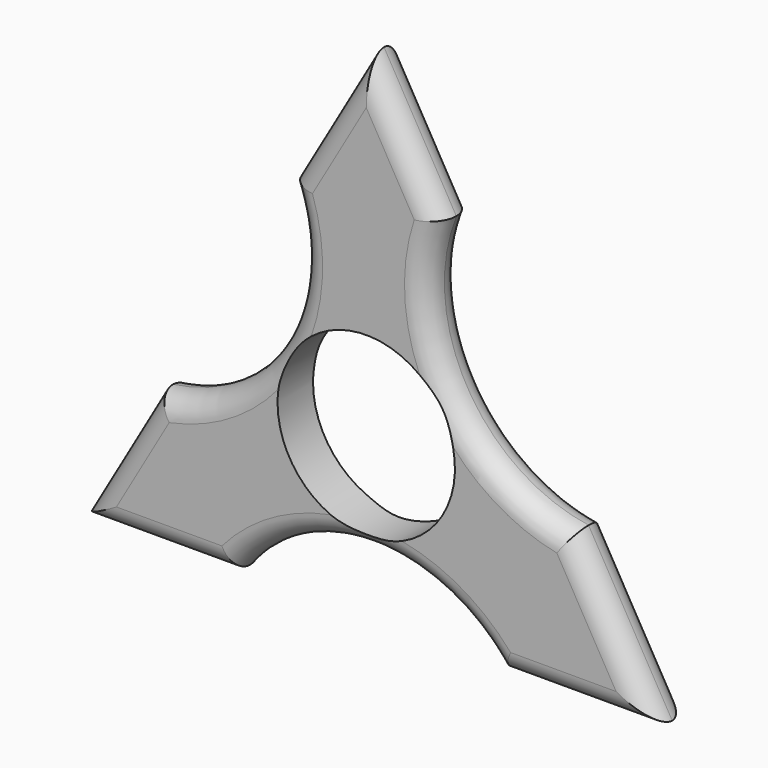
from build123d import *

# Parameters (mm, degrees)
F2_DEPTH     = 5
F3_D         = 20
F5_DEPTH     = 5
F7_T1_DEPTH  = 28.8144071543
F7_T3_DEPTH  = 30.1295341717
F7_T5_DEPTH  = 31.3559112982
F7_T7_DEPTH  = 29.9091460928
F7_T9_DEPTH  = 29.9091460928
F7_T11_DEPTH = 29.9018260823
F7_T14_ANGLE = 141.1544022781
F7_T16_ANGLE = 142.8852494642
F7_T18_ANGLE = 141.8336244917
F7_T20_ANGLE = 141.8336244917
F7_T22_ANGLE = 141.1544022781
F7_T24_ANGLE = 142.8852494642


# Not quite as in the source:
# - a fillet or chamfer that OpenCascade refuses, or shapes differently, is made with other operations: its cross-section is extruded or revolved along the edge and cut away or added
# - a feature of the source that left no trace in its solid (it failed there, or was rolled back) is left out


with BuildPart() as f2:
    # F0 (on Front) → F2 (new body)
    with BuildSketch(Plane.XZ):
        Polygon((0, 56.291651246), (-32.5, 0), (32.5, 0), align=None)
    extrude(amount=F2_DEPTH)

    # F3 (through all)
    with Locations(Plane(origin=(0, 0, 0), x_dir=(1, 0, 0), z_dir=(0, 1, 0))):
        with Locations((0, -18.7304634601)):
            Hole(F3_D / 2)

    # F4 (on face) → F5 (cut)
    with BuildSketch(Plane.XZ.offset(5)):
        with BuildLine():
            Line((-8.8147670858, 41.0240267964), (-23.7990869589, 15.0704234595))
            ThreePointArc((-23.7990869589, 15.0704234595), (-9.9693914422, 24.3882472548), (-8.8147670858, 41.0240267964))
        make_face()
        with BuildLine():
            Line((23.0720443509, 16.3296981957), (8.1572035772, 42.1629602027))
            ThreePointArc((8.1572035772, 42.1629602027), (9.353798316, 25.631639826), (23.0720443509, 16.3296981957))
        make_face()
        with BuildLine():
            ThreePointArc((15.0908539072, 0), (0, 7.455905044), (-15.0908539072, 0))
            Line((-15.0908539072, 0), (15.0908539072, 0))
        make_face()
    extrude(amount=-F5_DEPTH, mode=Mode.SUBTRACT)

    # F7: fillet of radius 2.5 on 18 edges, made by hand

    # F7_s2 → F7_t1 (cut)
    with BuildSketch(Plane(origin=(-13.0927964228, 0, 22.6773886175), x_dir=(0, 1, 0), z_dir=(-0.5, 0, 0.8660254038))):
        with BuildLine():
            ThreePointArc((0, -25.645825623), (-0.732233047, -27.413592576), (-2.5, -28.145825623))
            Line((-2.5, -28.145825623), (0, -28.145825623))
            Line((0, -28.145825623), (0, -25.645825623))
        make_face()
        with BuildLine():
            ThreePointArc((-5, -25.645825623), (-4.267766953, -27.413592576), (-2.5, -28.145825623))
            Line((-2.5, -28.145825623), (-5, -28.145825623))
            Line((-5, -28.145825623), (-5, -25.645825623))
        make_face()
    extrude(amount=F7_T1_DEPTH, mode=Mode.SUBTRACT)

    # F7_s4 → F7_t3 (cut)
    with BuildSketch(Plane(origin=(27.5, 0, 47.6313972081), x_dir=(0, 1, 0), z_dir=(-0.5, 0, -0.8660254038))):
        with BuildLine():
            ThreePointArc((-2.5, -28.145825623), (-0.732233047, -27.413592576), (0, -25.645825623))
            Line((0, -25.645825623), (0, -28.145825623))
            Line((0, -28.145825623), (-2.5, -28.145825623))
        make_face()
        with BuildLine():
            ThreePointArc((-2.5, -28.145825623), (-4.267766953, -27.413592576), (-5, -25.645825623))
            Line((-5, -25.645825623), (-5, -28.145825623))
            Line((-5, -28.145825623), (-2.5, -28.145825623))
        make_face()
    extrude(amount=F7_T3_DEPTH, mode=Mode.SUBTRACT)

    # F7_s6 → F7_t5 (cut)
    with BuildSketch(Plane(origin=(11.25, 0, -19.4855715851), x_dir=(0, 1, 0), z_dir=(-0.5, 0, 0.8660254038))):
        with BuildLine():
            ThreePointArc((0, -25.645825623), (-0.732233047, -27.413592576), (-2.5, -28.145825623))
            Line((-2.5, -28.145825623), (0, -28.145825623))
            Line((0, -28.145825623), (0, -25.645825623))
        make_face()
        with BuildLine():
            ThreePointArc((-5, -25.645825623), (-4.267766953, -27.413592576), (-2.5, -28.145825623))
            Line((-2.5, -28.145825623), (-5, -28.145825623))
            Line((-5, -28.145825623), (-5, -25.645825623))
        make_face()
    extrude(amount=F7_T5_DEPTH, mode=Mode.SUBTRACT)

    # F7_s8 → F7_t7 (cut)
    with BuildSketch(Plane.YZ.offset(8.8408539072)):
        with BuildLine():
            ThreePointArc((0, 2.5), (-0.732233047, 0.732233047), (-2.5, 0))
            Line((-2.5, 0), (0, 0))
            Line((0, 0), (0, 2.5))
        make_face()
        with BuildLine():
            ThreePointArc((-5, 2.5), (-4.267766953, 0.732233047), (-2.5, 0))
            Line((-2.5, 0), (-5, 0))
            Line((-5, 0), (-5, 2.5))
        make_face()
    extrude(amount=F7_T7_DEPTH, mode=Mode.SUBTRACT)

    # F7_s10 → F7_t9 (cut)
    with BuildSketch(Plane.YZ.offset(-38.75)):
        with BuildLine():
            ThreePointArc((0, 2.5), (-0.732233047, 0.732233047), (-2.5, 0))
            Line((-2.5, 0), (0, 0))
            Line((0, 0), (0, 2.5))
        make_face()
        with BuildLine():
            ThreePointArc((-5, 2.5), (-4.267766953, 0.732233047), (-2.5, 0))
            Line((-2.5, 0), (-5, 0))
            Line((-5, 0), (-5, 2.5))
        make_face()
    extrude(amount=F7_T9_DEPTH, mode=Mode.SUBTRACT)

    # F7_s12 → F7_t11 (cut)
    with BuildSketch(Plane(origin=(3.7009130411, 0, 6.4101694217), x_dir=(0, 1, 0), z_dir=(-0.5, 0, -0.8660254038))):
        with BuildLine():
            ThreePointArc((0, -25.645825623), (-0.732233047, -27.413592576), (-2.5, -28.145825623))
            Line((-2.5, -28.145825623), (0, -28.145825623))
            Line((0, -28.145825623), (0, -25.645825623))
        make_face()
        with BuildLine():
            ThreePointArc((-5, -25.645825623), (-4.267766953, -27.413592576), (-2.5, -28.145825623))
            Line((-2.5, -28.145825623), (-5, -28.145825623))
            Line((-5, -28.145825623), (-5, -25.645825623))
        make_face()
    extrude(amount=F7_T11_DEPTH, mode=Mode.SUBTRACT)

    # F7_s13 → F7_t14 (revolve, cut)
    with BuildSketch(Plane(origin=(28.2767394092, 0, 33.0176183098), x_dir=(0, 1, 0), z_dir=(0.6504720402, 0, 0.7595302002))):
        with BuildLine():
            ThreePointArc((0, 24.7499806074), (-0.732233047, 22.9822136544), (-2.5, 22.2499806074))
            Line((-2.5, 22.2499806074), (0, 22.2499806074))
            Line((0, 22.2499806074), (0, 24.7499806074))
        make_face()
    revolve(axis=Axis((25.8082809879, 0, 35.131639826), (0, -1, 0)), revolution_arc=F7_T14_ANGLE, mode=Mode.SUBTRACT)

    # F7_s15 → F7_t16 (revolve, cut)
    with BuildSketch(Plane(origin=(3.4829302285, 0, -10.374843271), x_dir=(0, 1, 0), z_dir=(0.3182541365, 0, -0.9480054349))):
        with BuildLine():
            ThreePointArc((0, 17.8260440287), (-0.732233047, 16.0582770757), (-2.5, 15.3260440287))
            Line((-2.5, 15.3260440287), (0, 15.3260440287))
            Line((0, 15.3260440287), (0, 17.8260440287))
        make_face()
    revolve(axis=Axis((0, 0, -11.544094956), (0, -1, 0)), revolution_arc=F7_T16_ANGLE, mode=Mode.SUBTRACT)

    # F7_s17 → F7_t18 (revolve, cut)
    with BuildSketch(Plane(origin=(-31.7778859418, 0, 6.129127173), x_dir=(0, 1, 0), z_dir=(-0.9819031843, 0, 0.1893835701))):
        with BuildLine():
            ThreePointArc((0, -6.7707302764), (-0.732233047, -8.5384972294), (-2.5, -9.2707302764))
            Line((-2.5, -9.2707302764), (0, -9.2707302764))
            Line((0, -9.2707302764), (0, -6.7707302764))
        make_face()
    revolve(axis=Axis((-26.4238741141, 0, 33.8882472548), (0, -1, 0)), revolution_arc=F7_T18_ANGLE, mode=Mode.SUBTRACT)

    # F7_s19 → F7_t20 (revolve, cut)
    with BuildSketch(Plane(origin=(-31.7778859418, 0, 6.129127173), x_dir=(0, 1, 0), z_dir=(-0.9819031843, 0, 0.1893835701))):
        with BuildLine():
            ThreePointArc((-2.5, -9.2707302764), (-4.267766953, -8.5384972294), (-5, -6.7707302764))
            Line((-5, -6.7707302764), (-5, -9.2707302764))
            Line((-5, -9.2707302764), (-2.5, -9.2707302764))
        make_face()
    revolve(axis=Axis((-26.4238741141, -5, 33.8882472548), (0, -1, 0)), revolution_arc=F7_T20_ANGLE, mode=Mode.SUBTRACT)

    # F7_s21 → F7_t22 (revolve, cut)
    with BuildSketch(Plane(origin=(28.2767394092, 0, 33.0176183098), x_dir=(0, 1, 0), z_dir=(0.6504720402, 0, 0.7595302002))):
        with BuildLine():
            ThreePointArc((-5, 24.7499806074), (-4.267766953, 22.9822136544), (-2.5, 22.2499806074))
            Line((-2.5, 22.2499806074), (-5, 22.2499806074))
            Line((-5, 22.2499806074), (-5, 24.7499806074))
        make_face()
    revolve(axis=Axis((25.8082809879, -5, 35.131639826), (0, -1, 0)), revolution_arc=F7_T22_ANGLE, mode=Mode.SUBTRACT)

    # F7_s23 → F7_t24 (revolve, cut)
    with BuildSketch(Plane(origin=(3.4829302285, 0, -10.374843271), x_dir=(0, 1, 0), z_dir=(0.3182541365, 0, -0.9480054349))):
        with BuildLine():
            ThreePointArc((-5, 17.8260440287), (-4.267766953, 16.0582770757), (-2.5, 15.3260440287))
            Line((-2.5, 15.3260440287), (-5, 15.3260440287))
            Line((-5, 15.3260440287), (-5, 17.8260440287))
        make_face()
    revolve(axis=Axis((0, -5, -11.544094956), (0, -1, 0)), revolution_arc=F7_T24_ANGLE, mode=Mode.SUBTRACT)


solid = f2.part
